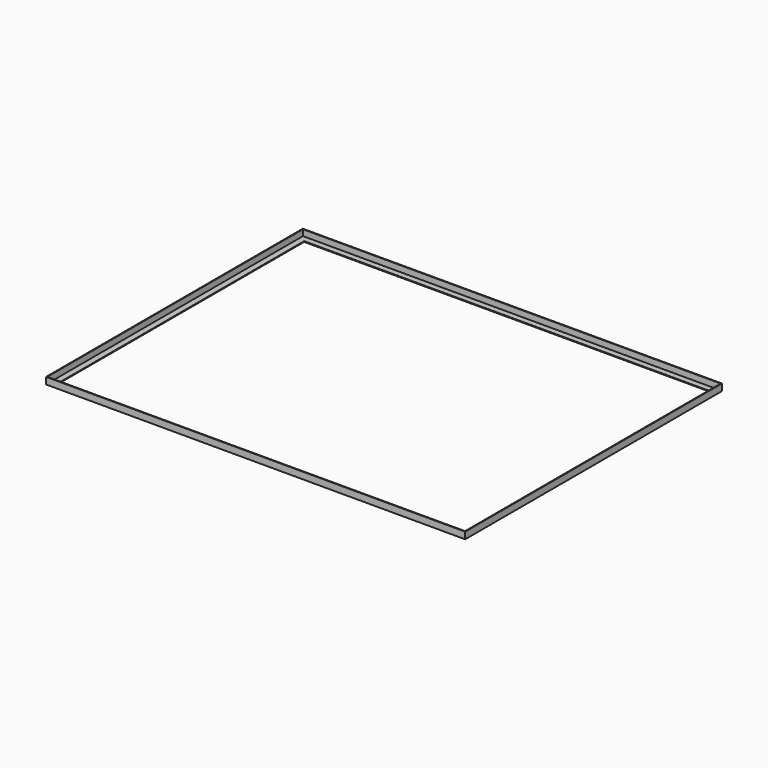
from build123d import *


with BuildPart() as f2:
    # F2: sweep along a path in F0
    with BuildLine(Plane.XY) as f2_path:
        Line((-373.5, 286), (-373.5, -286))
        Line((-373.5, -286), (373.5, -286))
        Line((373.5, -286), (373.5, 286))
        Line((373.5, 286), (-373.5, 286))
    # F1 (on Front) → F2 (sweep)
    with BuildSketch(Plane.XZ):
        Polygon((-372.3, 12), (-373.5, 12), (-373.5, 0), (-361.5, 0), (-361.5, 1.2), (-372.3, 1.2), align=None)
    sweep(path=f2_path.line, transition=Transition.RIGHT)


solid = f2.part
